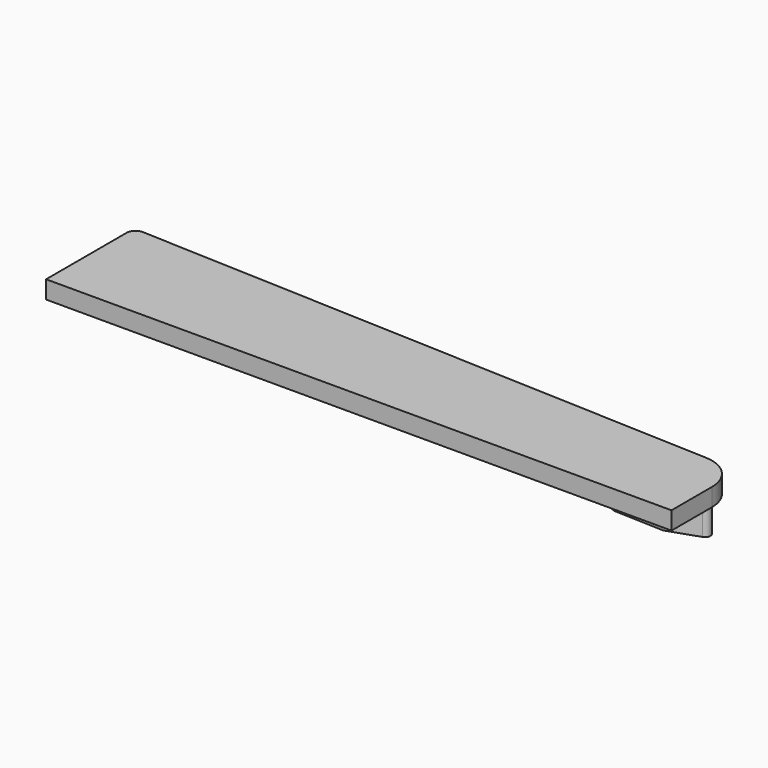
from build123d import *

# Parameters (mm, degrees)
F1_DEPTH = 2
F3_DEPTH = 7
F4_R     = 0.6
F5_R     = 4
F6_R     = 1


# Not quite as in the source:
# - a feature of the source that left no trace in its solid (it failed there, or was rolled back) is left out


with BuildPart() as f1:
    # F0 (on Top) → F1 (new body)
    with BuildSketch(Plane.XY):
        Polygon((0, 12.3), (0, 0), (70, 0), (70, 9.5), align=None)
    extrude(amount=F1_DEPTH)

    # F2 (on face) → F3 (join)
    with BuildSketch(Plane.XY.offset(2)):
        Polygon((1, 11.8), (1, 8.8), (7.8769936128, 8.5249202555), (10.9920095872, 11.4003196165), align=None)
        Polygon((63.4, 7.0580007994), (69.9, 9.3), (49.9159808256, 10.099360767), (57.8044746312, 7.2818218141), align=None)
    extrude(amount=-F3_DEPTH)

    # F4
    f4_edges = [f1.edges().sort_by_distance(p)[0] for p in [
        (1, 11.8, -2.5),
        (10.99201, 11.40032, -2.5),
        (69.9, 9.3, -2.5),
        (49.915981, 10.099361, -2.5),
        (63.4, 7.058001, -2.5),
        (57.804475, 7.281822, -2.5),
        (1, 8.8, -2.5),
        (7.876994, 8.52492, -2.5),
    ]]
    fillet(f4_edges, radius=F4_R)

    # F5
    f5_edges = [f1.edges().sort_by_distance(p)[0] for p in [
        (70, 9.5, 1),
    ]]
    fillet(f5_edges, radius=F5_R)

    # F6
    f6_edges = [f1.edges().sort_by_distance(p)[0] for p in [
        (0, 12.3, 1),
    ]]
    fillet(f6_edges, radius=F6_R)


solid = f1.part
